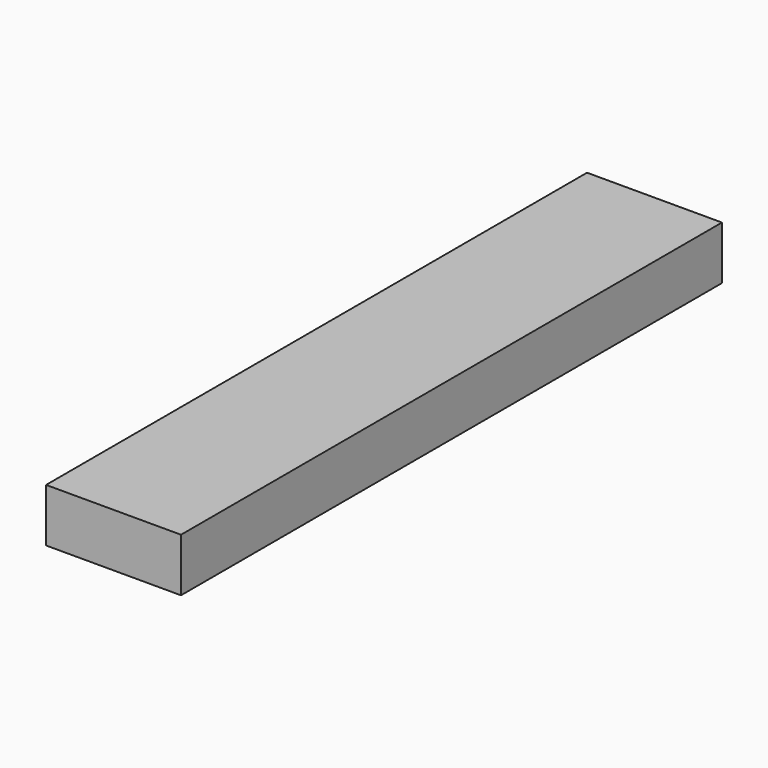
from build123d import *

# Parameters (mm, degrees)
F0_W     = 21.8460857868
F0_H     = 109.4911545515
F1_DEPTH = 8.6363647133


# Not quite as in the source:
# - the program builds the solid bodies; features that only make, move or delete a surface that nothing else refers to are left out


with BuildPart() as f1:
    # F0 (on Top) → F1 (new body)
    with BuildSketch(Plane.XY):
        with Locations((0, -54.7455772758)):
            Rectangle(F0_W, F0_H)
    extrude(amount=F1_DEPTH)


solid = f1.part
